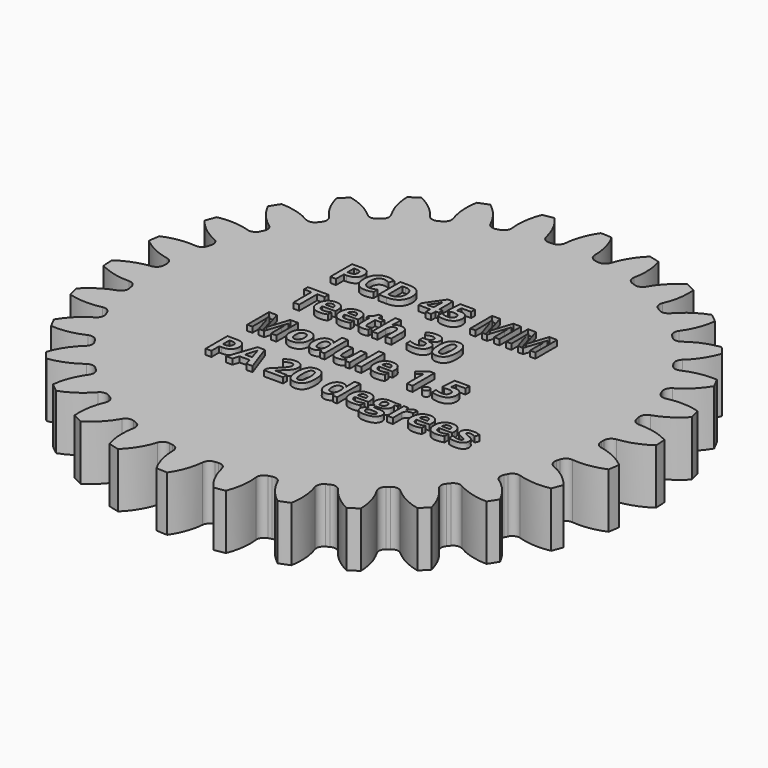
from build123d import *

# Parameters (mm, degrees)
F1_DEPTH     = 5
F2_R         = 0.673469388
F3_COUNT     = 30
F4_TEXT_SIZE = 3.4722222222
F5_DEPTH     = 0.5


# Not quite as in the source:
# - Text() gives the source's letters only with a copy of the font that has no kerning and outlines rounded to 1/6400 em; it was checked with that copy


with BuildPart() as f1:
    # F0 (on Top) → F1 (new body)
    with BuildSketch(Plane.XY):
        with BuildLine():
            ThreePointArc((-0.5009671403, 20.6189150278), (-14.4058699448, -14.7601333373), (20.625, 0))
            ThreePointArc((20.625, 0), (15.3668259328, 13.7568632235), (2.2733601697, 20.499328246))
            ThreePointArc((2.2733601697, 20.499328246), (0.8882114119, 20.6058658029), (-0.5009671403, 20.6189150278))
        make_face()
        with BuildLine():
            ThreePointArc((-0.5009671403, 20.6189150278), (0.8882114119, 20.6058658029), (2.2733601697, 20.499328246))
            ThreePointArc((2.2733601697, 20.499328246), (2.1707292524, 22.2805149081), (1.5424740436, 23.9503814964))
            ThreePointArc((1.5424740436, 23.9503814964), (1.0335550975, 23.9777347525), (0.5241700707, 23.9942752701))
            ThreePointArc((0.5241700707, 23.9942752701), (-0.2454463413, 22.3846636372), (-0.5009671403, 20.6189150278))
        make_face()
    extrude(amount=F1_DEPTH)

    # F2
    f2_edges = [f1.edges().sort_by_distance(p)[0] for p in [
        (-0.500967, 20.618915, 2.5),
        (2.27336, 20.499328, 2.5),
    ]]
    fillet(f2_edges, radius=F2_R)

    # F3: F1 ×30 about axis
    f3_axis = Axis((0, 0, 0), (0, 0, -1))


with BuildPart() as f1_1:
    add(f1.part)
    for i in range(1, F3_COUNT):
        add(f1.part.rotate(f3_axis, i * 360 / F3_COUNT))

    # F4 (on face) → F5 (join)
    with BuildSketch(Plane.XY.offset(5)):
        with Locations((-10, 6)):
            Text('PCD 45 MM', F4_TEXT_SIZE, font='Open Sans', font_style=FontStyle.BOLD, text_align=(TextAlign.LEFT, TextAlign.BOTTOM))
        with Locations((-10, 1.2777777778)):
            Text('Teeth 30', F4_TEXT_SIZE, font='Open Sans', font_style=FontStyle.BOLD, text_align=(TextAlign.LEFT, TextAlign.BOTTOM))
        with Locations((-10, -3.4444444444)):
            Text('Module 1.5', F4_TEXT_SIZE, font='Open Sans', font_style=FontStyle.BOLD, text_align=(TextAlign.LEFT, TextAlign.BOTTOM))
        with Locations((-10, -8.1666666667)):
            Text('PA 20 degrees', F4_TEXT_SIZE, font='Open Sans', font_style=FontStyle.BOLD, text_align=(TextAlign.LEFT, TextAlign.BOTTOM))
    extrude(amount=F5_DEPTH)


solid = f1_1.part
